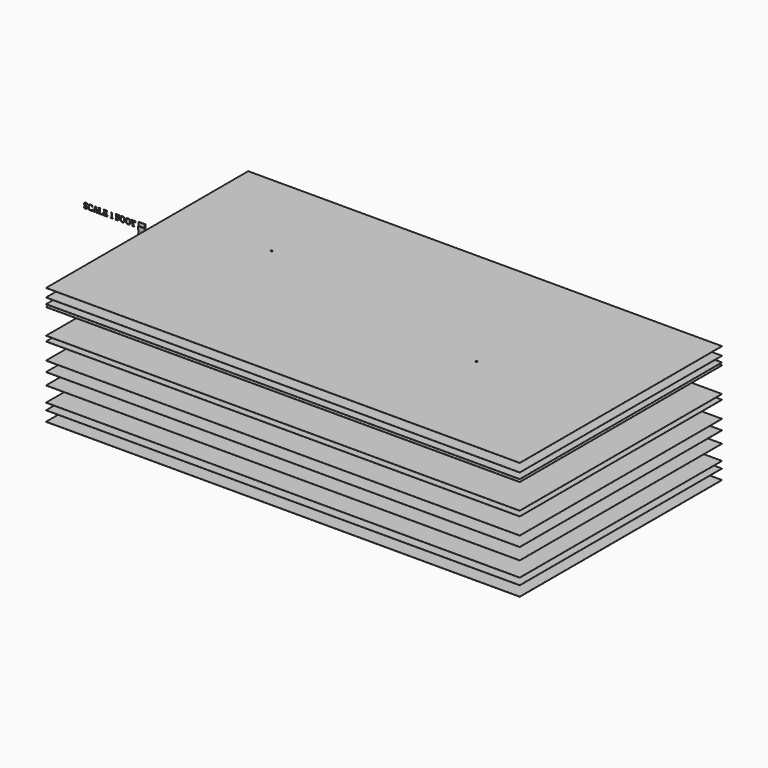
from build123d import *

# Parameters (mm, degrees)
F0_W          = 42892.5876617432
F0_H          = 22882.0877075195
F1_DEPTH      = 12.7
F13_R         = 76.2
F14_DEPTH     = 10680.701
F16_TEXT_SIZE = 693.4698257181
F17_DEPTH     = 30.48
F15_W         = 609.6
F15_H         = 304.8
F18_DEPTH     = 30.48
F15_H_2       = 304.8000000001
F15_H_3       = 304.8000000002
F19_DEPTH     = 91.44


# Not quite as in the source:
# - Text() gives the source's letters only with a copy of the font that has no kerning and outlines rounded to 1/6400 em; it was checked with that copy


with BuildPart() as f1:
    # F0 (on Top) → F1 (new body)
    with BuildSketch(Plane.XY):
        with Locations((7855.7195663452, -571.0048675537)):
            Rectangle(F0_W, F0_H)
    extrude(amount=F1_DEPTH)


with BuildPart() as f2_1:
    # F2: copy of F1
    add(f1.part.moved(Location((0, 0, -762))))


with BuildPart() as f3_1:
    # F3: copy of F1
    add(f1.part.moved(Location((0, 0, -1295.4))))


with BuildPart() as f4_1:
    # F4: copy of F1
    add(f1.part.moved(Location((0, 0, -1524))))


with BuildPart() as f5_1:
    # F5: copy of F1
    add(f1.part.moved(Location((0, 0, -3810))))


with BuildPart() as f6_1:
    # F6: copy of F1
    add(f1.part.moved(Location((0, 0, -4267.2))))


with BuildPart() as f7_1:
    # F7: copy of F1
    add(f1.part.moved(Location((0, 0, -5791.2))))


with BuildPart() as f8_1:
    # F8: copy of F1
    add(f1.part.moved(Location((0, 0, -6705.6))))


with BuildPart() as f9_1:
    # F9: copy of F1
    add(f1.part.moved(Location((0, 0, -7772.4))))


with BuildPart() as f10_1:
    # F10: copy of F1
    add(f1.part.moved(Location((0, 0, -9144))))


with BuildPart() as f11_1:
    # F11: copy of F1
    add(f1.part.moved(Location((0, 0, -9753.6))))


with BuildPart() as f12_1:
    # F12: copy of F1
    add(f1.part.moved(Location((0, 0, -10668))))


with BuildPart() as f14_tool:
    # F13 (on face) → F14 (new body, through all)
    with BuildSketch(Plane.XY.offset(12.7)):
        with Locations((-4667.5219535828, 2370.0187206268)):
            Circle(F13_R)
        with Locations((17228.5003662109, -1797.3231077194)):
            Circle(F13_R)
    extrude(amount=-F14_DEPTH)


with BuildPart() as f1_1:
    add(f1.part)

    # F14: cut by f14_tool
    add(f14_tool.part, mode=Mode.SUBTRACT)


with BuildPart() as f2_1_1:
    add(f2_1.part)

    # F14: cut by f14_tool
    add(f14_tool.part, mode=Mode.SUBTRACT)


with BuildPart() as f3_1_1:
    add(f3_1.part)

    # F14: cut by f14_tool
    add(f14_tool.part, mode=Mode.SUBTRACT)


with BuildPart() as f4_1_1:
    add(f4_1.part)

    # F14: cut by f14_tool
    add(f14_tool.part, mode=Mode.SUBTRACT)


with BuildPart() as f5_1_1:
    add(f5_1.part)

    # F14: cut by f14_tool
    add(f14_tool.part, mode=Mode.SUBTRACT)


with BuildPart() as f6_1_1:
    add(f6_1.part)

    # F14: cut by f14_tool
    add(f14_tool.part, mode=Mode.SUBTRACT)


with BuildPart() as f7_1_1:
    add(f7_1.part)

    # F14: cut by f14_tool
    add(f14_tool.part, mode=Mode.SUBTRACT)


with BuildPart() as f8_1_1:
    add(f8_1.part)

    # F14: cut by f14_tool
    add(f14_tool.part, mode=Mode.SUBTRACT)


with BuildPart() as f9_1_1:
    add(f9_1.part)

    # F14: cut by f14_tool
    add(f14_tool.part, mode=Mode.SUBTRACT)


with BuildPart() as f10_1_1:
    add(f10_1.part)

    # F14: cut by f14_tool
    add(f14_tool.part, mode=Mode.SUBTRACT)


with BuildPart() as f11_1_1:
    add(f11_1.part)

    # F14: cut by f14_tool
    add(f14_tool.part, mode=Mode.SUBTRACT)


with BuildPart() as f12_1_1:
    add(f12_1.part)

    # F14: cut by f14_tool
    add(f14_tool.part, mode=Mode.SUBTRACT)


with BuildPart() as f17:
    # F16 (on Front) → F17 (new body)
    with BuildSketch(Plane.XZ):
        with Locations((-19795.5637040626, -499.2982745171)):
            Text('SCALE 1 FOOT', F16_TEXT_SIZE, font='Tinos', text_align=(TextAlign.LEFT, TextAlign.BOTTOM))
    extrude(amount=F17_DEPTH)


with BuildPart() as f18:
    # F15 (on Front) → F18 (new body)
    with BuildSketch(Plane.XZ):
        with Locations((-14504.9742645264, -152.4)):
            Rectangle(F15_W, F15_H)
    extrude(amount=F18_DEPTH)


with BuildPart() as f18b:
    # F15 (on Front) → F18, piece 2 (new body)
    with BuildSketch(Plane.XZ):
        with Locations((-14504.9742645264, -762)):
            Rectangle(F15_W, F15_H)
    extrude(amount=F18_DEPTH)


with BuildPart() as f18c:
    # F15 (on Front) → F18, piece 3 (new body)
    with BuildSketch(Plane.XZ):
        with Locations((-14504.9742645264, -1371.6)):
            Rectangle(F15_W, F15_H)
    extrude(amount=F18_DEPTH)


with BuildPart() as f18d:
    # F15 (on Front) → F18, piece 4 (new body)
    with BuildSketch(Plane.XZ):
        with Locations((-14504.9742645264, -1981.2)):
            Rectangle(F15_W, F15_H)
    extrude(amount=F18_DEPTH)


with BuildPart() as f18e:
    # F15 (on Front) → F18, piece 5 (new body)
    with BuildSketch(Plane.XZ):
        with Locations((-14504.9742645264, -2590.8)):
            Rectangle(F15_W, F15_H)
    extrude(amount=F18_DEPTH)


with BuildPart() as f18f:
    # F15 (on Front) → F18, piece 6 (new body)
    with BuildSketch(Plane.XZ):
        with Locations((-14504.9742645264, -3200.4)):
            Rectangle(F15_W, F15_H)
    extrude(amount=F18_DEPTH)


with BuildPart() as f18g:
    # F15 (on Front) → F18, piece 7 (new body)
    with BuildSketch(Plane.XZ):
        with Locations((-14504.9742645264, -3810)):
            Rectangle(F15_W, F15_H)
    extrude(amount=F18_DEPTH)


with BuildPart() as f18h:
    # F15 (on Front) → F18, piece 8 (new body)
    with BuildSketch(Plane.XZ):
        with Locations((-14504.9742645264, -4419.6)):
            Rectangle(F15_W, F15_H)
    extrude(amount=F18_DEPTH)


with BuildPart() as f18i:
    # F15 (on Front) → F18, piece 9 (new body)
    with BuildSketch(Plane.XZ):
        with Locations((-14504.9742645264, -5029.1999999999)):
            Rectangle(F15_W, F15_H_2)
    extrude(amount=F18_DEPTH)


with BuildPart() as f18j:
    # F15 (on Front) → F18, piece 10 (new body)
    with BuildSketch(Plane.XZ):
        with Locations((-14504.9742645264, -5638.7999999999)):
            Rectangle(F15_W, F15_H_2)
    extrude(amount=F18_DEPTH)


with BuildPart() as f18k:
    # F15 (on Front) → F18, piece 11 (new body)
    with BuildSketch(Plane.XZ):
        with Locations((-14504.9742645264, -6248.3999999999)):
            Rectangle(F15_W, F15_H_2)
    extrude(amount=F18_DEPTH)


with BuildPart() as f18l:
    # F15 (on Front) → F18, piece 12 (new body)
    with BuildSketch(Plane.XZ):
        with Locations((-14504.9742645264, -6857.9999999999)):
            Rectangle(F15_W, F15_H_2)
    extrude(amount=F18_DEPTH)


with BuildPart() as f18m:
    # F15 (on Front) → F18, piece 13 (new body)
    with BuildSketch(Plane.XZ):
        with Locations((-14504.9742645264, -7467.5999999999)):
            Rectangle(F15_W, F15_H_3)
    extrude(amount=F18_DEPTH)


with BuildPart() as f18n:
    # F15 (on Front) → F18, piece 14 (new body)
    with BuildSketch(Plane.XZ):
        with Locations((-14504.9742645264, -8686.8)):
            Rectangle(F15_W, F15_H)
    extrude(amount=F18_DEPTH)


with BuildPart() as f18o:
    # F15 (on Front) → F18, piece 15 (new body)
    with BuildSketch(Plane.XZ):
        with Locations((-14504.9742645264, -8077.2)):
            Rectangle(F15_W, F15_H)
    extrude(amount=F18_DEPTH)


with BuildPart() as f18p:
    # F15 (on Front) → F18, piece 16 (new body)
    with BuildSketch(Plane.XZ):
        with Locations((-14504.9742645264, -9296.4)):
            Rectangle(F15_W, F15_H)
    extrude(amount=F18_DEPTH)


with BuildPart() as f18q:
    # F15 (on Front) → F18, piece 17 (new body)
    with BuildSketch(Plane.XZ):
        with Locations((-14504.9742645264, -9906)):
            Rectangle(F15_W, F15_H)
    extrude(amount=F18_DEPTH)


with BuildPart() as f18r:
    # F15 (on Front) → F18, piece 18 (new body)
    with BuildSketch(Plane.XZ):
        with Locations((-14504.9742645264, -10515.6)):
            Rectangle(F15_W, F15_H)
    extrude(amount=F18_DEPTH)


with BuildPart() as f19:
    # F15 (on Front) → F19 (new body)
    with BuildSketch(Plane.XZ):
        with Locations((-14504.9742645264, -457.2)):
            Rectangle(F15_W, F15_H)
    extrude(amount=F19_DEPTH)


with BuildPart() as f19b:
    # F15 (on Front) → F19, piece 2 (new body)
    with BuildSketch(Plane.XZ):
        with Locations((-14504.9742645264, -1066.8)):
            Rectangle(F15_W, F15_H)
    extrude(amount=F19_DEPTH)


with BuildPart() as f19c:
    # F15 (on Front) → F19, piece 3 (new body)
    with BuildSketch(Plane.XZ):
        with Locations((-14504.9742645264, -1676.4)):
            Rectangle(F15_W, F15_H)
    extrude(amount=F19_DEPTH)


with BuildPart() as f19d:
    # F15 (on Front) → F19, piece 4 (new body)
    with BuildSketch(Plane.XZ):
        with Locations((-14504.9742645264, -2286)):
            Rectangle(F15_W, F15_H)
    extrude(amount=F19_DEPTH)


with BuildPart() as f19e:
    # F15 (on Front) → F19, piece 5 (new body)
    with BuildSketch(Plane.XZ):
        with Locations((-14504.9742645264, -2895.6)):
            Rectangle(F15_W, F15_H)
    extrude(amount=F19_DEPTH)


with BuildPart() as f19f:
    # F15 (on Front) → F19, piece 6 (new body)
    with BuildSketch(Plane.XZ):
        with Locations((-14504.9742645264, -3505.2)):
            Rectangle(F15_W, F15_H)
    extrude(amount=F19_DEPTH)


with BuildPart() as f19g:
    # F15 (on Front) → F19, piece 7 (new body)
    with BuildSketch(Plane.XZ):
        with Locations((-14504.9742645264, -4114.8)):
            Rectangle(F15_W, F15_H)
    extrude(amount=F19_DEPTH)


with BuildPart() as f19h:
    # F15 (on Front) → F19, piece 8 (new body)
    with BuildSketch(Plane.XZ):
        with Locations((-14504.9742645264, -4724.4)):
            Rectangle(F15_W, F15_H)
    extrude(amount=F19_DEPTH)


with BuildPart() as f19i:
    # F15 (on Front) → F19, piece 9 (new body)
    with BuildSketch(Plane.XZ):
        with Locations((-14504.9742645264, -5333.9999999999)):
            Rectangle(F15_W, F15_H_2)
    extrude(amount=F19_DEPTH)


with BuildPart() as f19j:
    # F15 (on Front) → F19, piece 10 (new body)
    with BuildSketch(Plane.XZ):
        with Locations((-14504.9742645264, -5943.5999999999)):
            Rectangle(F15_W, F15_H_2)
    extrude(amount=F19_DEPTH)


with BuildPart() as f19k:
    # F15 (on Front) → F19, piece 11 (new body)
    with BuildSketch(Plane.XZ):
        with Locations((-14504.9742645264, -6553.1999999999)):
            Rectangle(F15_W, F15_H_2)
    extrude(amount=F19_DEPTH)


with BuildPart() as f19l:
    # F15 (on Front) → F19, piece 12 (new body)
    with BuildSketch(Plane.XZ):
        with Locations((-14504.9742645264, -7162.7999999999)):
            Rectangle(F15_W, F15_H_3)
    extrude(amount=F19_DEPTH)


with BuildPart() as f19m:
    # F15 (on Front) → F19, piece 13 (new body)
    with BuildSketch(Plane.XZ):
        with Locations((-14504.9742645264, -7772.3999999999)):
            Rectangle(F15_W, F15_H_3)
    extrude(amount=F19_DEPTH)


with BuildPart() as f19n:
    # F15 (on Front) → F19, piece 14 (new body)
    with BuildSketch(Plane.XZ):
        with Locations((-14504.9742645264, -8382)):
            Rectangle(F15_W, F15_H)
    extrude(amount=F19_DEPTH)


with BuildPart() as f19o:
    # F15 (on Front) → F19, piece 15 (new body)
    with BuildSketch(Plane.XZ):
        with Locations((-14504.9742645264, -8991.6)):
            Rectangle(F15_W, F15_H)
    extrude(amount=F19_DEPTH)


with BuildPart() as f19p:
    # F15 (on Front) → F19, piece 16 (new body)
    with BuildSketch(Plane.XZ):
        with Locations((-14504.9742645264, -9601.2)):
            Rectangle(F15_W, F15_H)
    extrude(amount=F19_DEPTH)


with BuildPart() as f19q:
    # F15 (on Front) → F19, piece 17 (new body)
    with BuildSketch(Plane.XZ):
        with Locations((-14504.9742645264, -10210.8)):
            Rectangle(F15_W, F15_H)
    extrude(amount=F19_DEPTH)


solid = Compound([f1_1.part, f2_1_1.part, f3_1_1.part, f4_1_1.part, f5_1_1.part, f6_1_1.part, f7_1_1.part, f8_1_1.part, f9_1_1.part, f10_1_1.part, f11_1_1.part, f12_1_1.part, f17.part, f18.part, f18b.part, f18c.part, f18d.part, f18e.part, f18f.part, f18g.part, f18h.part, f18i.part, f18j.part, f18k.part, f18l.part, f18m.part, f18n.part, f18o.part, f18p.part, f18q.part, f18r.part, f19.part, f19b.part, f19c.part, f19d.part, f19e.part, f19f.part, f19g.part, f19h.part, f19i.part, f19j.part, f19k.part, f19l.part, f19m.part, f19n.part, f19o.part, f19p.part, f19q.part])
